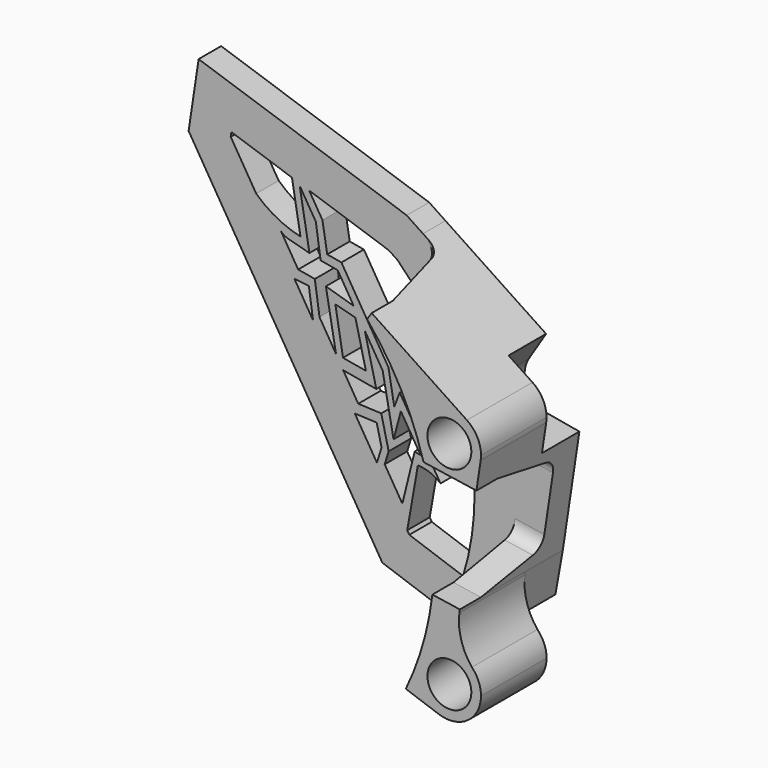
from build123d import *

# Parameters (mm, degrees)
F1_DEPTH = 6.096
F0_R     = 4.7625
F2_DEPTH = 27.94
F3_R     = 4.7625
F4_DEPTH = 10.16
F6_DEPTH = 25.4
F8_DEPTH = 25.4


# Not quite as in the source:
# - ends of sketch curves that miss each other by under 0.0002 mm in the source are joined


with BuildPart() as f1:
    # F0 (on Front) → F1 (new body)
    with BuildSketch(Plane.XZ):
        with BuildLine():
            Line((-32.0214776694, -42.0687062724), (-9.4581565389, -49.9383443038))
            ThreePointArc((-9.4581565389, -49.9383443038), (-4.3291887886, -10.8925785557), (-23.2082019061, 23.6683964993))
            Line((-23.2082019061, 23.6683964993), (-26.7419346225, 26.0181961702))
            Line((-26.7419346225, 26.0181961702), (-71.8849952467, 41.1920125155))
            Line((-71.8849952467, 41.1920125155), (-74.0636416555, 26.7504224083))
            Line((-74.0636416555, 26.7504224083), (-32.0214776694, -42.0687062724))
        make_face()
        with BuildLine():
            Line((-64.9229101249, 28.5970199237), (-64.7778869932, 29.5583345343))
            Line((-64.7778869932, 29.5583345343), (-51.6396961272, 25.1422295438))
            Line((-51.6396961272, 25.1422295438), (-52.8126453404, 31.9232999149))
            Line((-52.8126453404, 31.9232999149), (-47.9094184009, 23.888381259))
            Line((-47.9094184009, 23.888381259), (-30.6306738726, 18.0805230295))
            Line((-30.6306738726, 18.0805230295), (-28.7005674828, 16.7970746978))
            ThreePointArc((-28.7005674828, 16.7970746978), (-13.7073707997, -9.0370384003), (-14.5091616555, -38.895947921))
            Line((-14.5091616555, -38.895947921), (-26.1770067548, -34.8264354141))
            Line((-26.1770067548, -34.8264354141), (-26.621853962, -34.0982617358))
            Line((-26.621853962, -34.0982617358), (-26.6298627107, -34.143893025))
            Line((-26.6298627107, -34.143893025), (-33.2056261218, -23.3681886247))
            Line((-33.2056261218, -23.3681886247), (-33.1959865258, -23.3370155967))
            Line((-33.1959865258, -23.3370155967), (-37.9909119068, -15.4881668334))
            Line((-37.9909119068, -15.4881668334), (-38.0149602805, -15.4871320814))
            Line((-38.0149602805, -15.4871320814), (-47.058612277, -0.6672983188))
            Line((-47.058612277, -0.6672983188), (-47.0628196228, -0.6382941035))
            Line((-47.0628196228, -0.6382941035), (-51.126360936, 6.0133466785))
            Line((-51.126360936, 6.0133466785), (-51.1360904547, 6.0144657282))
            Line((-51.1360904547, 6.0144657282), (-59.3956089847, 19.549339872))
            Line((-59.3956089847, 19.549339872), (-64.9229101249, 28.5970199237))
        make_face(mode=Mode.SUBTRACT)
        Polygon((-52.8126453404, 31.9232999149), (-51.6396961272, 25.1422295438), (-47.9094184009, 23.888381259), align=None)
        with BuildLine():
            Line((-47.9094184009, 23.888381259), (-51.6396961272, 25.1422295438))
            Line((-51.6396961272, 25.1422295438), (-49.7922885775, 14.4619712189))
            ThreePointArc((-49.7922885775, 14.4619712189), (-54.9303785287, 16.3705840809), (-59.3956089847, 19.549339872))
            Line((-59.3956089847, 19.549339872), (-51.126360936, 6.0133466785))
            Line((-51.126360936, 6.0133466785), (-47.9751295821, 5.650904873))
            Line((-47.9751295821, 5.650904873), (-47.0628196228, -0.6382941035))
            Line((-47.0628196228, -0.6382941035), (-37.9909119068, -15.4881668334))
            Line((-37.9909119068, -15.4881668334), (-33.2459525636, -15.6923326562))
            Line((-33.2459525636, -15.6923326562), (-32.1973996311, -20.1077332485))
            Line((-32.1973996311, -20.1077332485), (-33.1959865258, -23.3370155967))
            Line((-33.1959865258, -23.3370155967), (-26.621853962, -34.0982617358))
            Line((-26.621853962, -34.0982617358), (-24.3119723824, -20.937295163))
            ThreePointArc((-24.3119723824, -20.937295163), (-21.7000142249, -21.4617233548), (-19.4071664649, -22.8182628838))
            Line((-19.4071664649, -22.8182628838), (-28.2510661679, -8.3257632317))
            Line((-28.2510661679, -8.3257632317), (-29.4364036114, -11.4075290833))
            Line((-29.4364036114, -11.4075290833), (-30.6980011467, -4.3159705476))
            Line((-30.6980011467, -4.3159705476), (-40.9051855797, 12.4105439777))
            Line((-40.9051855797, 12.4105439777), (-43.9856683867, 12.9511995939))
            Line((-43.9856683867, 12.9511995939), (-45.0197701825, 19.1531143287))
            Line((-45.0197701825, 19.1531143287), (-47.9094184009, 23.888381259))
        make_face()
        Polygon((-27.6263519566, -29.1291445767), (-27.7209985719, -29.3173462139), (-31.515369772, -23.0995096098), (-30.6589124026, -20.3298531285), (-32.2562875166, -13.6033915394), (-37.2546680921, -13.3883215232), (-40.5128122557, -8.0492002372), (-33.339172628, -9.3082459116), (-35.8258069544, 1.0090607264), (-31.9595713249, -5.326540128), (-29.5939579287, -17.6900622221), (-28.0038996356, -11.8086998658), (-23.7145710116, -18.8376232681), (-25.0080493325, -18.5184438136), align=None, mode=Mode.SUBTRACT)
        Polygon((-42.2277428728, 4.0048563327), (-37.873417838, 2.8701371118), (-35.5923646419, -6.559544504), (-40.5642118698, -5.6869354699), align=None, mode=Mode.SUBTRACT)
        with BuildLine():
            Line((-46.4479878328, 18.3739303005), (-45.4261892475, 11.3299486454))
            Line((-45.4261892475, 11.3299486454), (-41.7172805078, 10.6789979777))
            Line((-41.7172805078, 10.6789979777), (-38.2356426654, 4.9736375696))
            Line((-38.2356426654, 4.9736375696), (-44.2720463387, 6.7649825752))
            Line((-44.2720463387, 6.7649825752), (-42.0774568025, -5.4481170908))
            Line((-42.0774568025, -5.4481170908), (-45.6646201437, 0.4301679667))
            Line((-45.6646201437, 0.4301679667), (-46.6726678742, 7.3793552358))
            Line((-46.6726678742, 7.3793552358), (-50.293044526, 8.0147676345))
            Line((-50.293044526, 8.0147676345), (-53.9911477917, 14.0748499614))
            ThreePointArc((-53.9911477917, 14.0748499614), (-53.0287307311, 13.4025301345), (-51.9140375876, 13.0341285278))
            Line((-51.9140375876, 13.0341285278), (-47.8512962747, 11.9523388206))
            Line((-47.8512962747, 11.9523388206), (-49.9565863421, 24.1234711571))
            Line((-49.9565863421, 24.1234711571), (-46.4479878328, 18.3739303005))
        make_face(mode=Mode.SUBTRACT)
        Polygon((-37.9909119068, -15.4881668334), (-47.0628196228, -0.6382941035), (-47.058612277, -0.6672983188), (-38.0149602805, -15.4871320814), align=None)
        Polygon((-26.621853962, -34.0982617358), (-33.1959865258, -23.3370155967), (-33.2056261218, -23.3681886247), (-26.6298627107, -34.143893025), align=None)
        Polygon((-51.126360936, 6.0133466785), (-59.3956089847, 19.549339872), (-51.1360904547, 6.0144657282), align=None)
    extrude(amount=F1_DEPTH)

    # F0 (on Front) → F2 (join)
    with BuildSketch(Plane.XZ):
        with BuildLine():
            ThreePointArc((-2.2585047177, -52.4494397874), (-6.6570778662, -44.3261291668), (1.0230165746, -39.1927316018))
            Line((1.0230165746, -39.1927316018), (2.1631019861, -31.6354491837))
            ThreePointArc((2.1631019861, -31.6354491837), (2.210106245, -31.292191847), (2.2664563284, -30.9503444137))
            Line((2.2664563284, -30.9503444137), (6.781268444, -1.0230162708))
            ThreePointArc((6.781268444, -1.0230162708), (-6.2699855461, -2.7783889669), (3.7973937006, 5.7106886698))
            Line((3.7973937006, 5.7106886698), (-23.2082019061, 23.6683964993))
            ThreePointArc((-23.2082019061, 23.6683964993), (-4.3291887886, -10.8925785557), (-9.4581565389, -49.9383443038))
            Line((-9.4581565389, -49.9383443038), (-2.2585047177, -52.4494397874))
        make_face()
        with BuildLine():
            ThreePointArc((3.7973937006, 5.7106886698), (-6.2699855461, -2.7783889669), (6.781268444, -1.0230162708))
            ThreePointArc((6.781268444, -1.0230162708), (6.8387902069, -0.5129449342), (6.858, 0))
            ThreePointArc((6.858, 0), (6.0446128908, 3.239570805), (3.7973937006, 5.7106886698))
        make_face()
        Circle(F0_R, mode=Mode.SUBTRACT)
        with BuildLine():
            Line((2.1631019861, -31.6354491837), (1.0230165746, -39.1927316018))
            ThreePointArc((1.0230165746, -39.1927316018), (3.1078508959, -39.8606190362), (4.8759932113, -41.1514639241))
            ThreePointArc((4.8759932113, -41.1514639241), (2.5546345778, -36.6685406241), (2.1631019861, -31.6354491837))
        make_face()
        with BuildLine():
            ThreePointArc((4.8759932113, -41.1514639241), (3.1078508959, -39.8606190362), (1.0230165746, -39.1927316018))
            ThreePointArc((1.0230165746, -39.1927316018), (-6.6570778662, -44.3261291668), (-2.2585047177, -52.4494397874))
            ThreePointArc((-2.2585047177, -52.4494397874), (3.9713561063, -51.5651085374), (6.858, -45.974))
            ThreePointArc((6.858, -45.974), (6.3431744987, -43.3670283318), (4.8759932113, -41.1514639241))
        make_face()
        with BuildLine():
            ThreePointArc((0.7104281768, -41.2647858346), (3.6100429666, -42.8677166857), (4.7625, -45.974))
            ThreePointArc((4.7625, -45.974), (-3.6100429666, -49.0802833143), (0.7104281768, -41.2647858346))
        make_face(mode=Mode.SUBTRACT)
    extrude(amount=F2_DEPTH)

    # F3 (on face) → F4 (cut)
    with BuildSketch(Plane(origin=(0, 0, 0), x_dir=(-1, 0, 0), z_dir=(0, 1, 0))):
        with BuildLine():
            ThreePointArc((1.0479234506, -5.9407838449), (4.6212906458, -3.8774642509), (6.0325, 0))
            ThreePointArc((6.0325, 0), (5.7966808552, 1.6701937951), (5.1076604432, 3.2098070109))
            ThreePointArc((5.1076604432, 3.2098070109), (-5.5141755069, 2.4464105806), (1.0479234506, -5.9407838449))
        make_face()
        Circle(F3_R, mode=Mode.SUBTRACT)
        with BuildLine():
            ThreePointArc((1.0479234506, -5.9407838449), (-5.5141755069, 2.4464105806), (5.1076604432, 3.2098070109))
            Line((5.1076604432, 3.2098070109), (1.3747032796, 9.1499391047))
            Line((1.3747032796, 9.1499391047), (-3.7973937006, 5.7106886698))
            ThreePointArc((-3.7973937006, 5.7106886698), (-6.2699855461, 2.7783889669), (-6.781268444, -1.0230162708))
            Line((-6.781268444, -1.0230162708), (-5.8556681398, -7.158541587))
            Line((-5.8556681398, -7.158541587), (1.0479234506, -5.9407838449))
        make_face()
        with BuildLine():
            Line((-0.6517694903, -39.9768129276), (-2.2664563284, -30.9503444137))
            ThreePointArc((-2.2664563284, -30.9503444137), (-2.46420133, -36.3340905871), (-4.8759932113, -41.1514639241))
            ThreePointArc((-4.8759932113, -41.1514639241), (-5.7986098468, -49.6357329019), (2.2585047177, -52.4494397874))
            Line((2.2585047177, -52.4494397874), (6.4636236378, -50.9827778723))
            Line((6.4636236378, -50.9827778723), (5.5451457053, -48.3493768874))
            ThreePointArc((5.5451457053, -48.3493768874), (-4.8488389859, -49.5628461571), (-0.6517694903, -39.9768129276))
        make_face()
        with BuildLine():
            ThreePointArc((6.0325, -45.974), (4.0286012957, -41.483852135), (-0.6517694903, -39.9768129276))
            ThreePointArc((-0.6517694903, -39.9768129276), (-4.8488389859, -49.5628461571), (5.5451457053, -48.3493768874))
            ThreePointArc((5.5451457053, -48.3493768874), (5.9094055419, -47.1864283036), (6.0325, -45.974))
        make_face()
        with Locations((0, -45.974)):
            Circle(F3_R, mode=Mode.SUBTRACT)
        with Locations((0, -45.974)):
            Circle(F3_R)
    extrude(amount=-F4_DEPTH, mode=Mode.SUBTRACT)

    # F5 (on face) → F6 (cut)
    with BuildSketch(Plane(origin=(6.7812683982, 0, -1.0230165746), x_dir=(0, 1, 0), z_dir=(0.9888113733, 0, -0.1491712707))):
        with BuildLine():
            Line((-27.94, -6.1359623937), (-27.94, -30.2659623937))
            Line((-27.94, -30.2659623937), (-22.225, -30.2659623937))
            Line((-22.225, -30.2659623937), (-8.6577684612, -27.5952475238))
            ThreePointArc((-8.6577684612, -27.5952475238), (-6.81869138, -26.496664003), (-6.096, -24.4800313066))
            Line((-6.096, -24.4800313066), (-6.096, -18.2009623937))
            Line((-6.096, -18.2009623937), (-6.096, -11.9218934807))
            ThreePointArc((-6.096, -11.9218934807), (-6.81869138, -9.9052607843), (-8.6577684612, -8.8066772635))
            Line((-8.6577684612, -8.8066772635), (-22.225, -6.1359623937))
            Line((-22.225, -6.1359623937), (-27.94, -6.1359623937))
        make_face()
    extrude(amount=-F6_DEPTH, mode=Mode.SUBTRACT)

    # F7 (on face) → F8 (cut)
    with BuildSketch(Plane(origin=(3.7973937006, 0, 5.7106886698), x_dir=(0.8327046763, 0, -0.5537173667), z_dir=(0.5537173667, 0, 0.8327046763))):
        with BuildLine():
            Line((-32.4311804374, -6.096), (-32.4311804374, -27.94))
            Line((-32.4311804374, -27.94), (-24.8111804374, -27.94))
            Line((-24.8111804374, -27.94), (-24.8111804374, -22.225))
            Line((-24.8111804374, -22.225), (-27.8331080585, -8.5842698128))
            ThreePointArc((-27.8331080585, -8.5842698128), (-28.9454580871, -6.7950160194), (-30.9329510626, -6.096))
            Line((-30.9329510626, -6.096), (-32.4311804374, -6.096))
        make_face()
    extrude(amount=-F8_DEPTH, mode=Mode.SUBTRACT)


solid = f1.part
